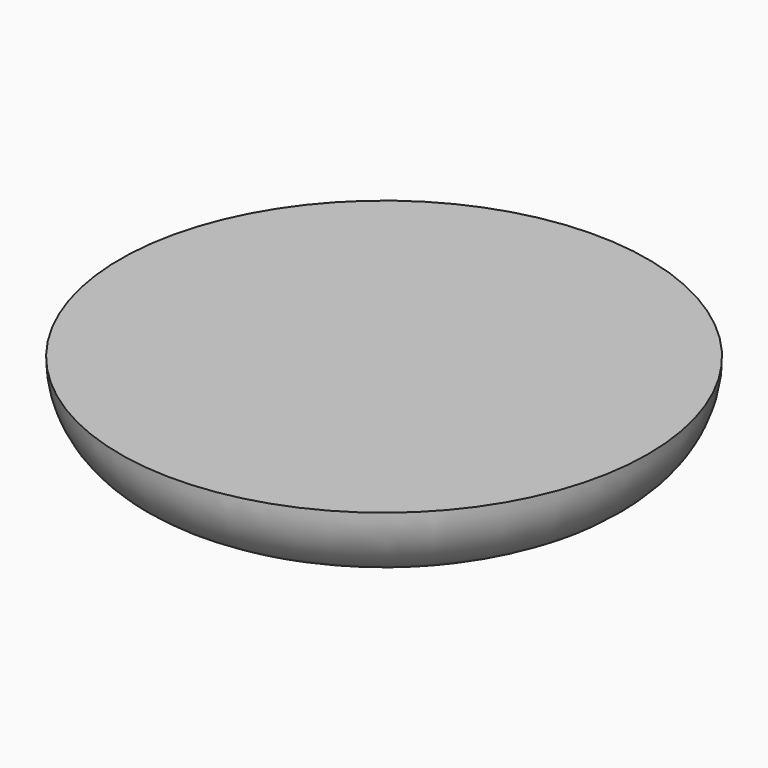
from build123d import *

# Parameters (mm, degrees)
F0_R     = 25.4
F1_DEPTH = 7.62
F2_R     = 7.61999


# Not quite as in the source:
# - a fillet or chamfer is up to 0.001 mm smaller than in the source, because OpenCascade refuses the exact size


with BuildPart() as f1:
    # F0 (on Top) → F1 (new body)
    with BuildSketch(Plane.XY):
        Circle(F0_R)
    extrude(amount=F1_DEPTH)

    # F2 (radius 7.62 in the source; OpenCascade refuses exactly that, so slightly less here)
    f2_edges = [f1.edges().sort_by_distance(p)[0] for p in [
        (-25.4, 0, 0),
    ]]
    fillet(f2_edges, radius=F2_R)


solid = f1.part
